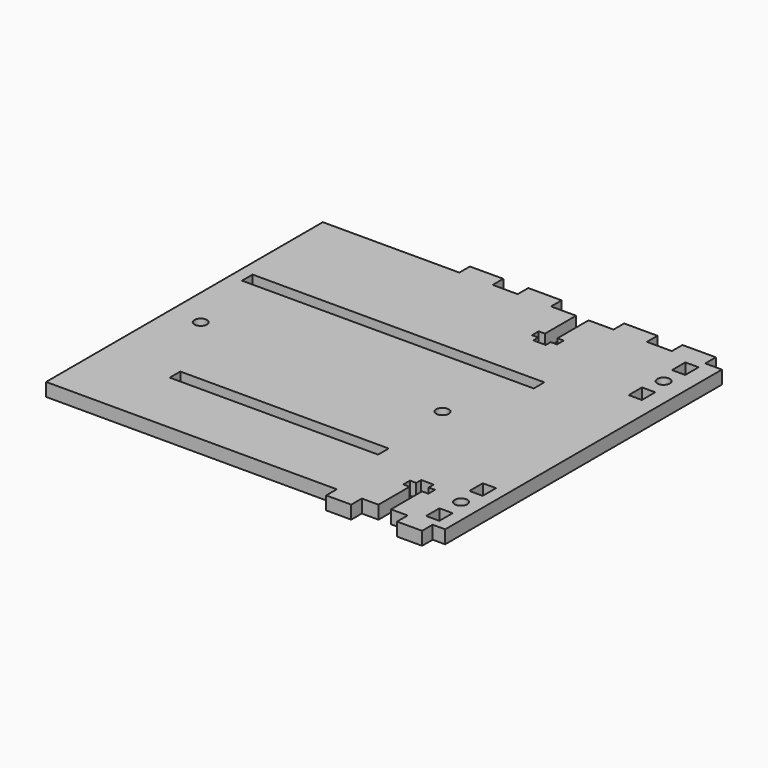
from build123d import *

# Parameters (mm, degrees)
F0_W     = 50
F0_H     = 3.175
F0_R     = 1.5
F0_W_2   = 3.175
F0_H_2   = 4
F0_W_3   = 70
F1_DEPTH = 3.175


# Not quite as in the source:
# - a length typed as a fraction of an inch, garbled in the dataset ("3 / 203.2 mm" for 3/8 in), is restored
# - a feature names something its author has since deleted; it is built from what else it names


with BuildPart() as f1:
    # F0 (on Top) → F1 (new body)
    with BuildSketch(Plane.XY):
        Polygon((46.1903014183, 27.8874409974), (43.1903014183, 27.8874409974), (43.1903014183, 29.3874409974), (41.6903014183, 29.3874409974), (41.6903014183, 31.3874409974), (43.1903014183, 31.3874409974), (43.1903014183, 40.7124409974), (37.1903014183, 40.7124409974), (37.1903014183, 43.8874409974), (29.1903014183, 43.8874409974), (29.1903014183, 40.7124409974), (23.1903014183, 40.7124409974), (23.1903014183, 43.8874409974), (15.1903014183, 43.8874409974), (15.1903014183, 40.7124409974), (-17.5596985817, 40.7124409974), (-17.5596985817, -42.2875590026), (52.1903014183, -42.2875590026), (52.1903014183, -45.4625590026), (58.1903014183, -45.4625590026), (58.1903014183, -42.2875590026), (62.1903014183, -42.2875590026), (62.1903014183, -32.9625590026), (60.6903014183, -32.9625590026), (60.6903014183, -30.9625590026), (62.1903014183, -30.9625590026), (62.1903014183, -29.4625590026), (65.1903014183, -29.4625590026), (65.1903014183, -30.9625590026), (66.6903014183, -30.9625590026), (66.6903014183, -32.9625590026), (65.1903014183, -32.9625590026), (65.1903014183, -42.2875590026), (69.1903014183, -42.2875590026), (69.1903014183, -45.4625590026), (75.1903014183, -45.4625590026), (75.1903014183, -42.2875590026), (78.1903014183, -42.2875590026), (78.1903014183, 40.7124409974), (74.1903014183, 40.7124409974), (74.1903014183, 43.8874409974), (66.1903014183, 43.8874409974), (66.1903014183, 40.7124409974), (60.1903014183, 40.7124409974), (60.1903014183, 43.8874409974), (52.1903014183, 43.8874409974), (52.1903014183, 40.7124409974), (46.1903014183, 40.7124409974), (46.1903014183, 31.3874409974), (47.6903014183, 31.3874409974), (47.6903014183, 29.3874409974), (46.1903014183, 29.3874409974), align=None)
        with Locations((24.4403014183, -24.8750590026)):
            Rectangle(F0_W, F0_H, mode=Mode.SUBTRACT)
        with Locations((-10.0596985817, -5.2875590026)):
            Circle(F0_R, mode=Mode.SUBTRACT)
        with Locations((73.6028014183, -38.2875590026)):
            Rectangle(F0_W_2, F0_H_2, mode=Mode.SUBTRACT)
        with Locations((73.6028014183, -31.7875590026)):
            Circle(F0_R, mode=Mode.SUBTRACT)
        with Locations((73.6028014183, -25.2875590026)):
            Rectangle(F0_W_2, F0_H_2, mode=Mode.SUBTRACT)
        with Locations((47.9403014183, -5.2875590026)):
            Circle(F0_R, mode=Mode.SUBTRACT)
        with Locations((20.4403014183, 14.2999409974)):
            Rectangle(F0_W_3, F0_H, mode=Mode.SUBTRACT)
        with Locations((72.6028014183, 23.7124409974)):
            Rectangle(F0_W_2, F0_H_2, mode=Mode.SUBTRACT)
        with Locations((72.6028014183, 30.2124409974)):
            Circle(F0_R, mode=Mode.SUBTRACT)
        with Locations((72.6028014183, 36.7124409974)):
            Rectangle(F0_W_2, F0_H_2, mode=Mode.SUBTRACT)
    extrude(amount=F1_DEPTH)


solid = f1.part
